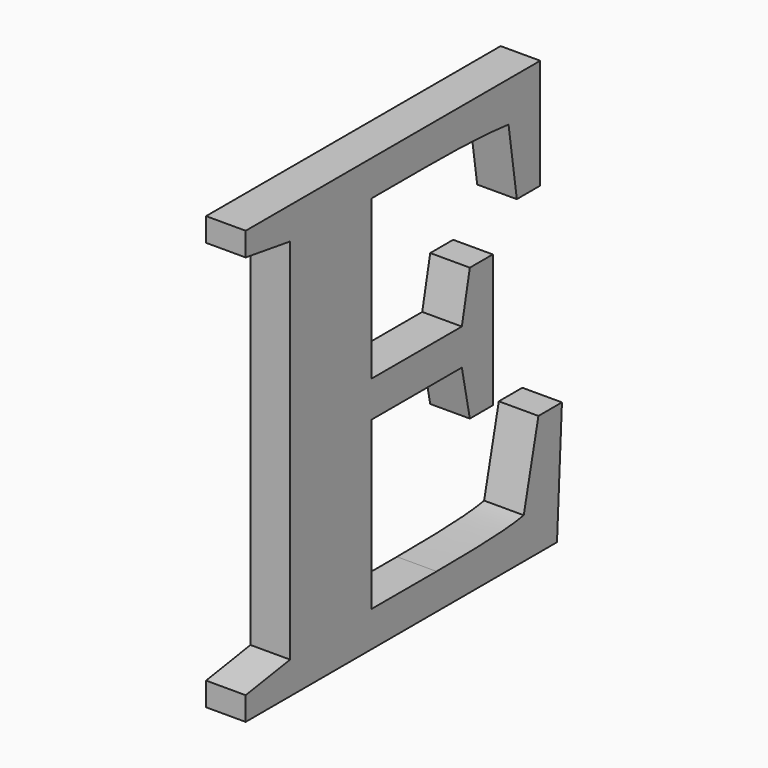
from build123d import *

# Parameters (mm, degrees)
F0_TEXT_SIZE = 635
F1_DEPTH     = 38.1


# Not quite as in the source:
# - Text() gives the source's letters only with a copy of the font that has no kerning and outlines rounded to 1/6400 em; it was checked with that copy


with BuildPart() as f1:
    # F0 (on Right) → F1 (new body)
    with BuildSketch(Plane.YZ):
        with Locations((-430.70859375, 0)):
            Text('E', F0_TEXT_SIZE, font='Tinos', font_style=FontStyle.BOLD, text_align=(TextAlign.LEFT, TextAlign.BOTTOM))
    extrude(amount=F1_DEPTH)


solid = f1.part
